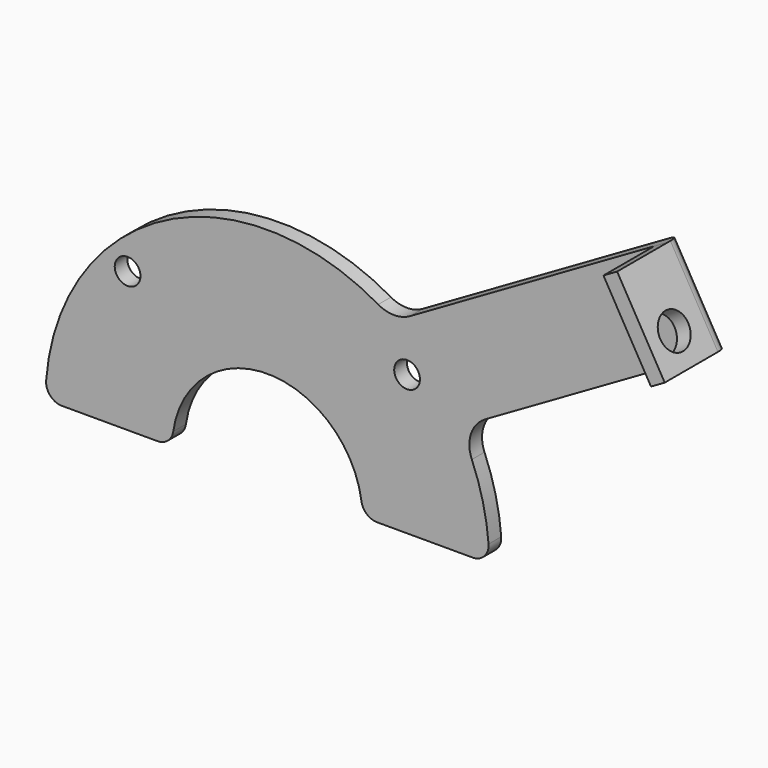
from build123d import *

# Parameters (mm, degrees)
F1_DEPTH = 6.35
F3_D     = 10.3124
F5_DEPTH = 25.4
F7_D     = 14
F8_R     = 12.7
F9_R     = 5.08
F10_R    = 6.35


# Not quite as in the source:
# - a feature names something its author has since deleted; it is built from what else it names


with BuildPart() as f1:
    # F0 (on Front) → F1 (new body)
    with BuildSketch(Plane.XZ):
        with BuildLine():
            Line((38.1, 0), (88.9, 0))
            ThreePointArc((88.9, 0), (85.8708059571, 23.0090131096), (76.9896583964, 44.45))
            Line((76.9896583964, 44.45), (179.5459910838, 103.6609262841))
            Line((179.5459910838, 103.6609262841), (160.4959910838, 136.6564941683))
            Line((160.4959910838, 136.6564941683), (50.5107648032, 73.1564941683))
            ThreePointArc((50.5107648032, 73.1564941683), (-41.3086129578, 78.7198100576), (-88.9, 0))
            Line((-88.9, 0), (-38.1, 0))
            ThreePointArc((-38.1, 0), (0, 38.1), (38.1, 0))
        make_face()
    extrude(amount=F1_DEPTH)

    # F3 (through all)
    with Locations(Plane.XZ.offset(6.35)):
        with Locations((-55.9918969149, 55.9918969149), (55.9918969149, 55.9918969149)):
            Hole(F3_D / 2)

    # F4 (on face) → F5 (join)
    with BuildSketch(Plane.XZ.offset(6.35)):
        Polygon((160.4959910838, 136.6564941683), (154.9967297697, 133.4814941683), (174.0467297697, 100.4859262841), (179.5459910838, 103.6609262841), align=None)
    extrude(amount=F5_DEPTH)

    # F7 (through all)
    with Locations(Plane(origin=(174.0467297697, 0, 100.4859262841), x_dir=(0, -1, 0), z_dir=(-0.8660254038, 0, -0.5))):
        with Locations((19.05, 12.7)):
            Hole(F7_D / 2)

    # F8
    f8_edges = [f1.edges().sort_by_distance(p)[0] for p in [
        (50.510765, -3.175, 73.156494),
        (76.989658, -3.175, 44.45),
    ]]
    fillet(f8_edges, radius=F8_R)

    # F9
    f9_edges = [f1.edges().sort_by_distance(p)[0] for p in [
        (170.020991, 0, 120.15871),
    ]]
    fillet(f9_edges, radius=F9_R)

    # F10
    f10_edges = [f1.edges().sort_by_distance(p)[0] for p in [
        (88.9, -3.175, 0),
        (38.1, -3.175, 0),
        (-38.1, -3.175, 0),
        (-88.9, -3.175, 0),
    ]]
    fillet(f10_edges, radius=F10_R)


solid = f1.part
